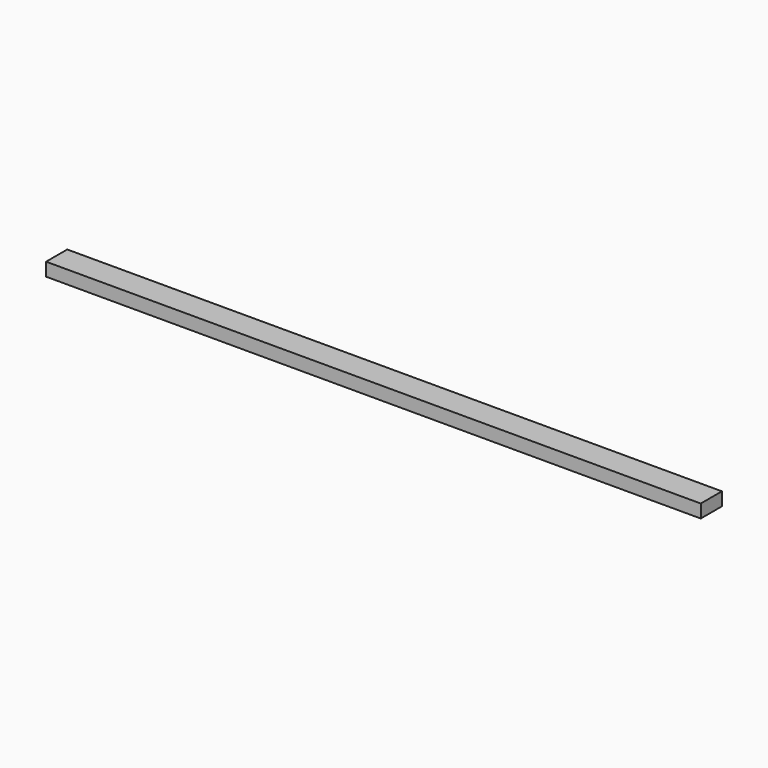
from build123d import *

# Parameters (mm, degrees)
F0_W     = 1257.3
F0_H     = 50.8
F1_DEPTH = 25.4


# Not quite as in the source:
# - a feature names something its author has since deleted; it is built from what else it names


with BuildPart() as f1:
    # F0 (on Top) → F1 (new body)
    with BuildSketch(Plane.XY):
        with Locations((628.65, 25.4)):
            Rectangle(F0_W, F0_H)
    extrude(amount=F1_DEPTH)


solid = f1.part
